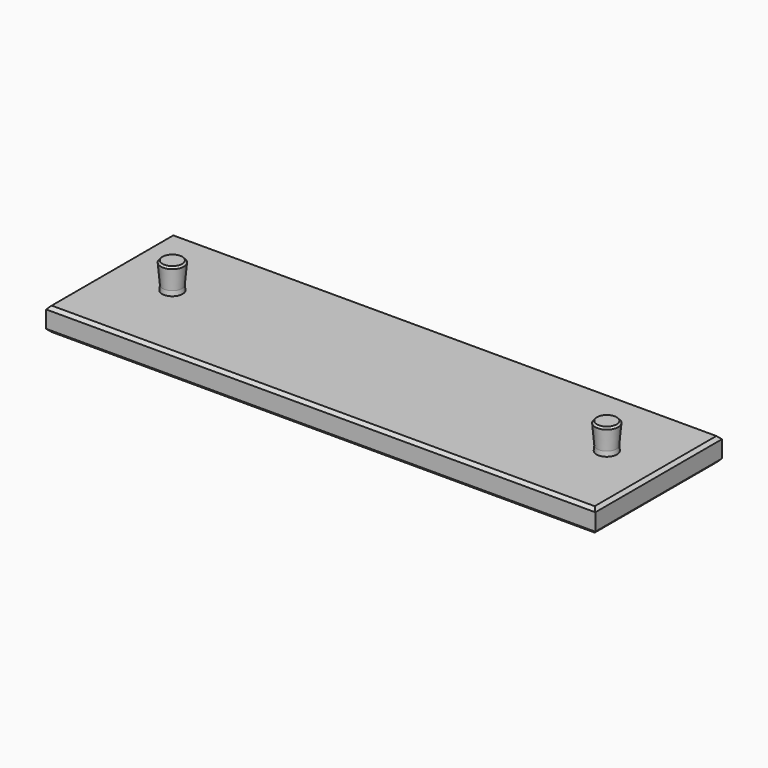
from build123d import *

# Parameters (mm, degrees)
F0_W      = 177
F0_H      = 51
F0_R      = 3.3
F1_DEPTH  = 7.5
F2_DEPTH  = 1.5
F2_TAPER  = 6
F2_FACE_R = 3.1423436471
F3_DEPTH  = 7
F3_TAPER  = -5
F5_SIZE   = 1


# Not quite as in the source:
# - a fillet or chamfer that OpenCascade refuses, or shapes differently, is made with other operations: its cross-section is extruded or revolved along the edge and cut away or added


with BuildPart() as f1:
    # F0 (on Top) → F1 (new body)
    with BuildSketch(Plane.XY):
        with Locations((-21.5246523023, -20.9546978474)):
            Rectangle(F0_W, F0_H)
        with Locations((-90.5246523023, -19.9546978474)):
            Circle(F0_R, mode=Mode.SUBTRACT)
        with Locations((49.4753476977, -19.9546978474)):
            Circle(F0_R, mode=Mode.SUBTRACT)
        with Locations((-90.5246523023, -19.9546978474)):
            Circle(F0_R)
        with Locations((49.4753476977, -19.9546978474)):
            Circle(F0_R)
    extrude(amount=-F1_DEPTH)

    # F0 (on Top) → F2 (join)
    with BuildSketch(Plane.XY):
        with Locations((-90.5246523023, -19.9546978474)):
            Circle(F0_R)
        with Locations((49.4753476977, -19.9546978474)):
            Circle(F0_R)
    extrude(amount=F2_DEPTH, taper=F2_TAPER)

    # F2_face (on face) → F3 (join)
    with BuildSketch(Plane(origin=(49.4753476977, -19.9546978474, 1.5), x_dir=(1, 0, 0), z_dir=(0, 0, 1))):
        Circle(F2_FACE_R)
        with Locations((-140, 0)):
            Circle(F2_FACE_R)
    extrude(amount=F3_DEPTH, taper=F3_TAPER)

    # F4: chamfer of 0.6 on 2 edges, made by hand

    # F4_s1 → F4_t2 (revolve, cut)
    with BuildSketch(Plane.XZ.offset(19.9546978474)):
        Polygon((-86.8221814561, 7.9022831811), (-87.3698880105, 8.5), (-86.7698880105, 8.5), align=None)
    revolve(axis=Axis((-90.5246523023, -19.9546978474, 8.5), (0, 0, -1)), mode=Mode.SUBTRACT)

    # F4_s3 → F4_t4 (revolve, cut)
    with BuildSketch(Plane.XZ.offset(19.9546978474)):
        Polygon((53.1778185439, 7.9022831811), (52.6301119895, 8.5), (53.2301119895, 8.5), align=None)
    revolve(axis=Axis((49.4753476977, -19.9546978474, 8.5), (0, 0, -1)), mode=Mode.SUBTRACT)

    # F5
    f5_edges = [f1.edges().sort_by_distance(p)[0] for p in [
        (-110.024652, -20.954698, 0),
        (-21.524652, 4.545302, 0),
        (-21.524652, -46.454698, 0),
        (66.975348, -20.954698, 0),
        (-21.524652, 4.545302, -7.5),
        (-110.024652, -20.954698, -7.5),
        (-21.524652, -46.454698, -7.5),
        (66.975348, -20.954698, -7.5),
    ]]
    chamfer(f5_edges, length=F5_SIZE)


solid = f1.part
